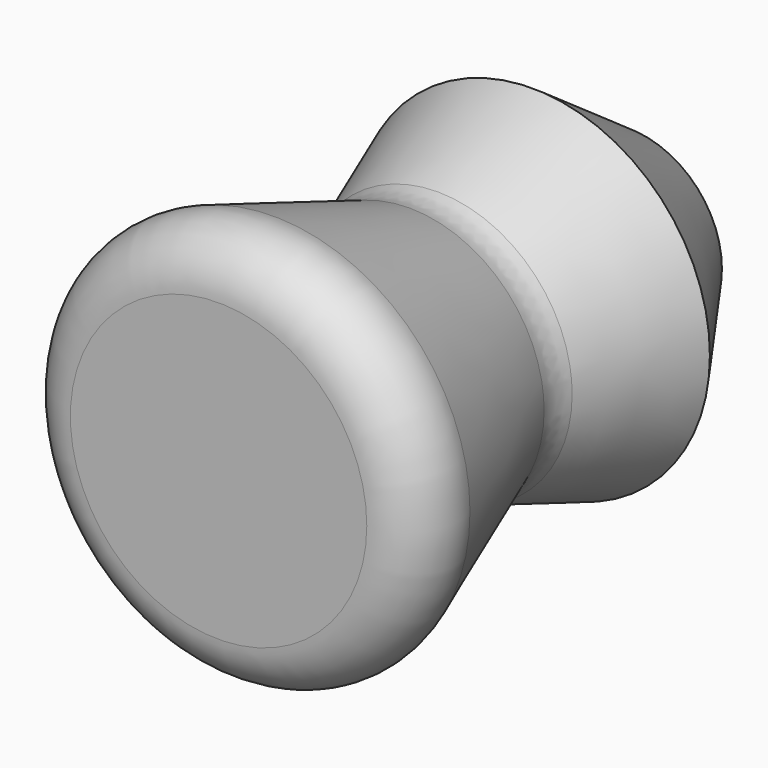
from build123d import *

# Parameters (mm, degrees)
F0_R     = 63.4990501998
F1_DEPTH = 127
F1_TAPER = -20
F2_R     = 25.4
F3_SIZE  = 63.5
F5_T     = -12.7


# Not quite as in the source:
# - a feature of the source that left no trace in its solid (it failed there, or was rolled back) is left out


with BuildPart() as f1:
    # F0 (on Front) → F1 (new body, symmetric)
    with BuildSketch(Plane.XZ):
        Circle(F0_R)
    extrude(amount=F1_DEPTH, both=True, taper=F1_TAPER)

    # F2
    f2_edges = [f1.edges().sort_by_distance(p)[0] for p in [
        (-63.49905, 0, 0),
        (-109.72327, -127, 0),
    ]]
    fillet(f2_edges, radius=F2_R)

    # F3
    f3_edges = [f1.edges().sort_by_distance(p)[0] for p in [
        (-109.72327, 127, 0),
    ]]
    chamfer(f3_edges, length=F3_SIZE)

    # F5
    f5_openings = [f1.faces().sort_by_distance(p)[0] for p in [
        (0, 127, 0),
    ]]
    offset(amount=F5_T, openings=f5_openings)


solid = f1.part
